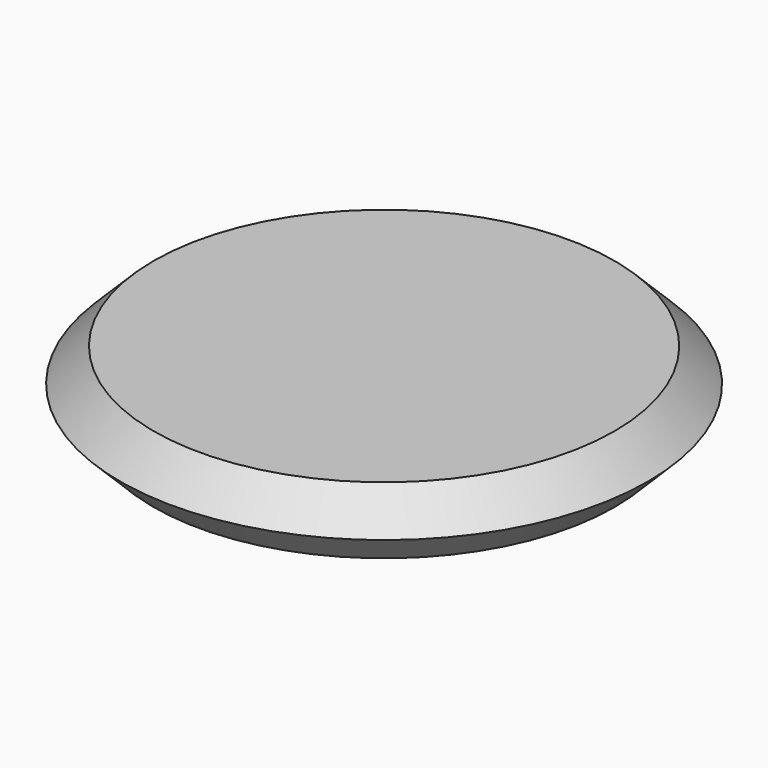
from build123d import *

# Parameters (mm, degrees)
F0_R     = 50.1004496622
F1_DEPTH = 12.7
F2_SIZE  = 6.35
F3_SIZE  = 6.34999


# Not quite as in the source:
# - a fillet or chamfer is up to 0.001 mm smaller than in the source, because OpenCascade refuses the exact size


with BuildPart() as f1:
    # F0 (on Top) → F1 (new body)
    with BuildSketch(Plane.XY):
        with Locations((-3.3122645349, -2.7786610853)):
            Circle(F0_R)
    extrude(amount=F1_DEPTH)

    # F2
    f2_edges = [f1.edges().sort_by_distance(p)[0] for p in [
        (-53.412714, -2.778661, 12.7),
    ]]
    chamfer(f2_edges, length=F2_SIZE)

    # F3 (size 6.35 in the source; OpenCascade refuses exactly that, so slightly less here)
    f3_edges = [f1.edges().sort_by_distance(p)[0] for p in [
        (-53.412714, -2.778661, 0),
    ]]
    chamfer(f3_edges, length=F3_SIZE)


solid = f1.part
